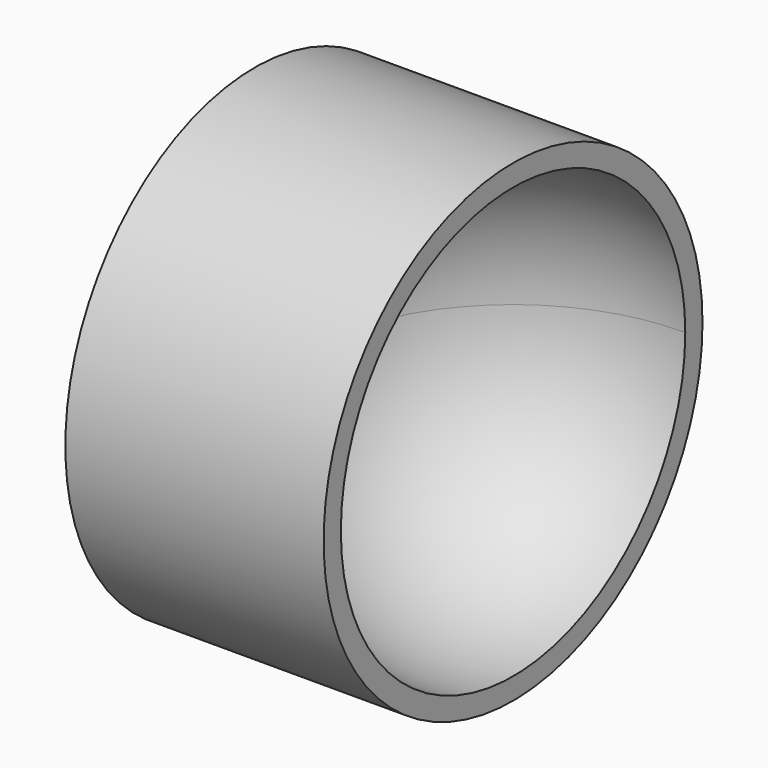
from build123d import *
from build123d import SkipClean  # not in build123d's __all__

# Parameters (mm, degrees)
F0_R     = 2.75
F1_DEPTH = 3


with BuildPart() as f1:
    # F0 (on Right) → F1 (new body)
    with BuildSketch(Plane.YZ):
        Circle(F0_R)
    extrude(amount=F1_DEPTH)

    # F2 (on Top) → F3 (revolve, cut)
    with BuildSketch(Plane.XY):
        with BuildLine():
            Line((3, -2.5), (3, 2.5))
            ThreePointArc((3, 2.5), (0.5, 0), (3, -2.5))
        make_face()
    with SkipClean():  # cleaning this boolean's faces spoils the solid; the shape is the same uncleaned
        revolve(axis=Axis((3, 0, 0), (0, -1, 0)), mode=Mode.SUBTRACT)


solid = f1.part
